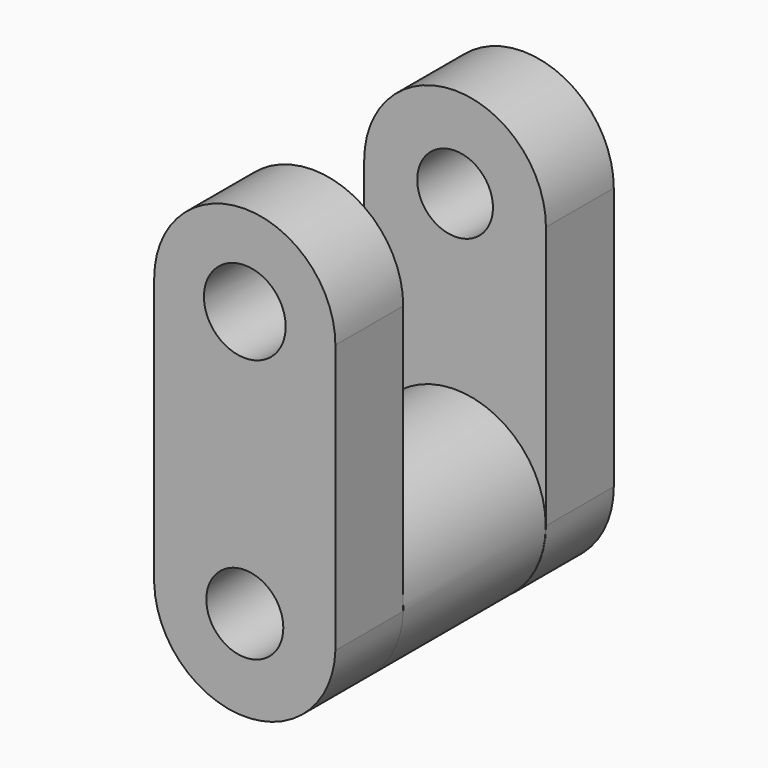
from build123d import *

# Parameters (mm, degrees)
F0_R     = 11.4715226447
F0_R_2   = 11.3474489307
F1_DEPTH = 25.4
F2_R     = 27.1514716213
F2_R_2   = 11.5339058998
F3_DEPTH = 53.34
F4_R     = 12.2446750111
F5_DEPTH = 25.4


with BuildPart() as f1:
    # F0 (on Front) → F1 (new body)
    with BuildSketch(Plane.XZ):
        with BuildLine():
            ThreePointArc((-27.219299227, -39.3772572279), (0, -12.1579580009), (27.219299227, -39.3772572279))
            Line((27.219299227, -39.3772572279), (27.219299227, 39.3772572279))
            ThreePointArc((27.219299227, 39.3772572279), (0, 12.1579580009), (-27.219299227, 39.3772572279))
            Line((-27.219299227, 39.3772572279), (-27.219299227, -39.3772572279))
        make_face()
        with BuildLine():
            ThreePointArc((-27.219299227, -39.3772572279), (0, -66.5965564549), (27.219299227, -39.3772572279))
            ThreePointArc((27.219299227, -39.3772572279), (0, -12.1579580009), (-27.219299227, -39.3772572279))
        make_face()
        with Locations((0, -39.3772572279)):
            Circle(F0_R, mode=Mode.SUBTRACT)
        with BuildLine():
            ThreePointArc((-27.219299227, 39.3772572279), (0, 12.1579580009), (27.219299227, 39.3772572279))
            ThreePointArc((27.219299227, 39.3772572279), (0, 66.5965564549), (-27.219299227, 39.3772572279))
        make_face()
        with Locations((0, 39.3772572279)):
            Circle(F0_R_2, mode=Mode.SUBTRACT)
    extrude(amount=F1_DEPTH)

    # F2 (on face) → F3 (join)
    with BuildSketch(Plane.XZ.offset(25.4)):
        with Locations((0, -39.3772572279)):
            Circle(F2_R)
        with Locations((0, -39.3772572279)):
            Circle(F2_R_2, mode=Mode.SUBTRACT)
    extrude(amount=F3_DEPTH)

    # F4 (on face) → F5 (join)
    with BuildSketch(Plane.XZ.offset(78.74)):
        with BuildLine():
            ThreePointArc((-27.1369592055, -40.2648699161), (0, -66.5287288492), (27.1369592055, -40.2648699161))
            Line((27.1369592055, -40.2648699161), (27.1369592055, -38.4896445397))
            ThreePointArc((27.1369592055, -38.4896445397), (0, -12.2257856066), (-27.1369592055, -38.4896445397))
            Line((-27.1369592055, -38.4896445397), (-27.1369592055, -40.2648699161))
        make_face()
        with BuildLine():
            ThreePointArc((4.719235111, -28.8530087858), (10.2659715637, -33.4010821613), (12.3491600723, -40.2648699161))
            ThreePointArc((12.3491600723, -40.2648699161), (-6.8637877548, -50.5308414798), (-4.719235111, -28.8530087858))
            ThreePointArc((-4.719235111, -28.8530087858), (0, -27.8433513281), (4.719235111, -28.8530087858))
        make_face(mode=Mode.SUBTRACT)
        with BuildLine():
            ThreePointArc((-27.1369592055, -38.4896445397), (0, -12.2257856066), (27.1369592055, -38.4896445397))
            Line((27.1369592055, -38.4896445397), (27.1369592055, 40.2648699161))
            ThreePointArc((27.1369592055, 40.2648699161), (0, 13.1279107106), (-27.1369592055, 40.2648699161))
            Line((-27.1369592055, 40.2648699161), (-27.1369592055, -38.4896445397))
        make_face()
        with BuildLine():
            ThreePointArc((-27.1369592055, 40.2648699161), (0, 13.1279107106), (27.1369592055, 40.2648699161))
            ThreePointArc((27.1369592055, 40.2648699161), (0, 67.4018291216), (-27.1369592055, 40.2648699161))
        make_face()
        with Locations((0, 40.2648699161)):
            Circle(F4_R, mode=Mode.SUBTRACT)
        with BuildLine():
            ThreePointArc((-4.719235111, -28.8530087858), (-6.8637877548, -50.5308414798), (12.3491600723, -40.2648699161))
            ThreePointArc((12.3491600723, -40.2648699161), (10.2659715637, -33.4010821613), (4.719235111, -28.8530087858))
            ThreePointArc((4.719235111, -28.8530087858), (9.6814822985, -33.1082951282), (11.5339058998, -39.3772572279))
            ThreePointArc((11.5339058998, -39.3772572279), (-6.2689620997, -49.0587395264), (-4.719235111, -28.8530087858))
        make_face()
    extrude(amount=F5_DEPTH)


solid = f1.part
